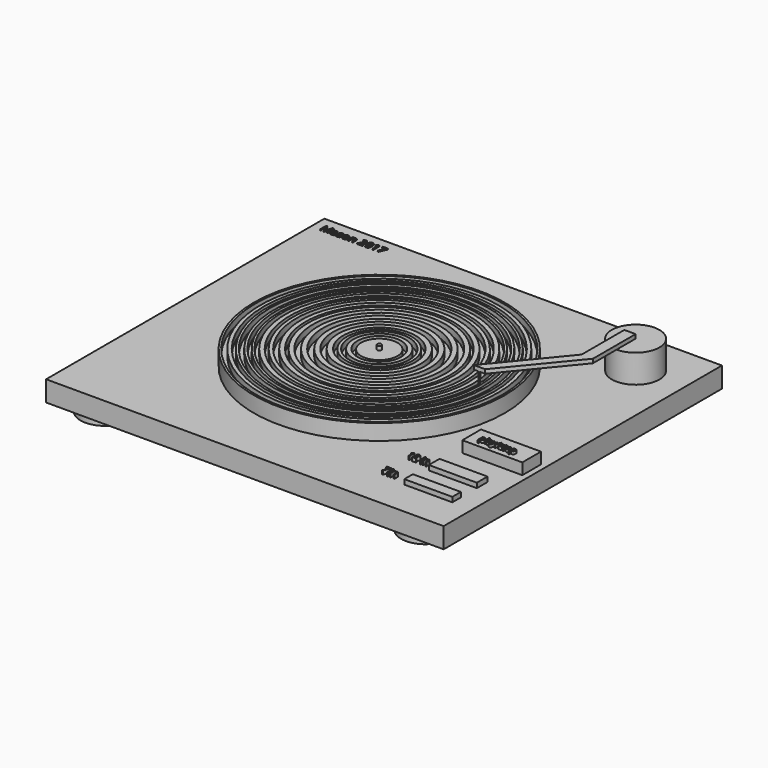
from build123d import *

# Parameters (mm, degrees)
F0_W            = 98.6984670162
F0_H            = 86.3612965102
F1_DEPTH        = 5.08
F2_R            = 31.156005255
F3_DEPTH        = 2.3
F4_R            = 31.156005255
F4_R_2          = 30.6611592983
F4_R_3          = 29.4866578201
F4_R_4          = 28.6056057905
F4_R_5          = 27.8142144613
F4_R_6          = 27.2510988872
F4_R_7          = 26.1923924199
F4_R_8          = 25.5781961877
F4_R_9          = 24.7586671221
F4_R_10         = 24.2262392051
F4_R_11         = 23.29553032
F4_R_12         = 22.2252370843
F4_R_13         = 21.4545488022
F4_R_14         = 20.5897211573
F4_R_15         = 19.4222273733
F4_R_16         = 18.2918713325
F4_R_17         = 17.6011317981
F4_R_18         = 16.4888289816
F4_R_19         = 15.1890669019
F4_R_20         = 13.9911540863
F4_R_21         = 12.6250610934
F4_R_22         = 11.4428912901
F4_R_23         = 10.2118226797
F4_R_24         = 8.9722442964
F4_R_25         = 8.1242020252
F4_R_26         = 7.4171270481
F4_R_27         = 6.4477778527
F4_R_28         = 5.420549124
F5_DEPTH        = 1.6
F6_R            = 5.9132088967
F7_DEPTH        = 7
F9_DEPTH        = 1
F11_DEPTH       = 0.4
F12_R           = 4.5011682677
F13_DEPTH       = 1.5
F14_R           = 0.5209758674
F15_DEPTH       = 1
F16_R           = 6
F17_DEPTH       = 2.6
F18_W           = 11.9140781462
F18_H           = 3.3094678074
F18_H_2         = 2.6475712657
F19_DEPTH       = 1.2
F20_TEXT_SIZE   = 2.5280596068
F20_TEXT_SIZE_2 = 2.2982376524
F21_DEPTH       = 0.9
F22_W           = 14.8925930262
F22_H           = 5.7915654033
F23_DEPTH       = 2.8
F24_TEXT_SIZE   = 2.0432040199
F25_DEPTH       = 0.7
F26_TEXT_SIZE   = 2.7578841481
F27_DEPTH       = 0.2


# Not quite as in the source:
# - Text() gives the source's letters only with a copy of the font that has no kerning and outlines rounded to 1/6400 em; it was checked with that copy


with BuildPart() as f1:
    # F0 (on Top) → F1 (new body)
    with BuildSketch(Plane.XY):
        with Locations((2.190053463, -1.2775995013)):
            Rectangle(F0_W, F0_H)
    extrude(amount=F1_DEPTH)

    # F2 (on face) → F3 (join)
    with BuildSketch(Plane.XY.offset(5.08)):
        Circle(F2_R)
    extrude(amount=F3_DEPTH)

    # F4 (on face) → F5 (join)
    with BuildSketch(Plane.XY.offset(7.38)):
        Circle(F4_R)
        Circle(F4_R_2, mode=Mode.SUBTRACT)
        Circle(F4_R_3)
        Circle(F4_R_4, mode=Mode.SUBTRACT)
        Circle(F4_R_5)
        Circle(F4_R_6, mode=Mode.SUBTRACT)
        Circle(F4_R_7)
        Circle(F4_R_8, mode=Mode.SUBTRACT)
        Circle(F4_R_9)
        Circle(F4_R_10, mode=Mode.SUBTRACT)
        Circle(F4_R_11)
        Circle(F4_R_12, mode=Mode.SUBTRACT)
        Circle(F4_R_13)
        Circle(F4_R_14, mode=Mode.SUBTRACT)
        Circle(F4_R_15)
        Circle(F4_R_16, mode=Mode.SUBTRACT)
        Circle(F4_R_17)
        Circle(F4_R_18, mode=Mode.SUBTRACT)
        Circle(F4_R_19)
        Circle(F4_R_20, mode=Mode.SUBTRACT)
        Circle(F4_R_21)
        Circle(F4_R_22, mode=Mode.SUBTRACT)
        Circle(F4_R_23)
        Circle(F4_R_24, mode=Mode.SUBTRACT)
        Circle(F4_R_25)
        Circle(F4_R_26, mode=Mode.SUBTRACT)
        Circle(F4_R_27)
        Circle(F4_R_28, mode=Mode.SUBTRACT)
    extrude(amount=F5_DEPTH)

    # F6 (on face) → F7 (join)
    with BuildSketch(Plane.XY.offset(5.08)):
        with Locations((39.8352257907, 29.7486409545)):
            Circle(F6_R)
    extrude(amount=F7_DEPTH)

    # F8 (on face) → F9 (join)
    with BuildSketch(Plane.XY.offset(12.08)):
        with BuildLine():
            Line((39.8352257907, 16.5107790381), (39.8352257907, 23.8354320578))
            ThreePointArc((39.8352257907, 23.8354320578), (38.3920917226, 24.0142357092), (37.0362326503, 24.5398333313))
            Line((37.0362326503, 24.5398333313), (37.0362326503, 16.5107790381))
            Line((37.0362326503, 16.5107790381), (23.4674233943, 0))
            Line((23.4674233943, 0), (26.2664165348, 0))
            Line((26.2664165348, 0), (39.8352257907, 16.5107790381))
        make_face()
        with BuildLine():
            Line((39.8352257907, 23.8354320578), (39.8352257907, 29.7486409545))
            Line((39.8352257907, 29.7486409545), (37.0362326503, 29.7486409545))
            Line((37.0362326503, 29.7486409545), (37.0362326503, 24.5398333313))
            ThreePointArc((37.0362326503, 24.5398333313), (38.3920917226, 24.0142357092), (39.8352257907, 23.8354320578))
        make_face()
    extrude(amount=F9_DEPTH)

    # F12 (on face) → F13 (join)
    with BuildSketch(Plane.XY.offset(7.38)):
        Circle(F12_R)
    extrude(amount=F13_DEPTH)

    # F14 (on face) → F15 (join)
    with BuildSketch(Plane.XY.offset(8.88)):
        Circle(F14_R)
    extrude(amount=F15_DEPTH)

    # F16 (on face) → F17 (join)
    with BuildSketch(Plane(origin=(0, 0, 0), x_dir=(1, 0, 0), z_dir=(0, 0, -1))):
        with Locations((-39.0016975826, 36.4318301551)):
            Circle(F16_R)
        with Locations((40.5705314347, 36.4318301551)):
            Circle(F16_R)
        with Locations((40.5705314347, -31.0741129819)):
            Circle(F16_R)
        with Locations((-39.0016975826, -32.8677496754)):
            Circle(F16_R)
    extrude(amount=F17_DEPTH)

    # F18 (on face) → F19 (join)
    with BuildSketch(Plane.XY.offset(5.08)):
        with Locations((40.6625922769, -26.3468036428)):
            Rectangle(F18_W, F18_H)
        with Locations((40.6625922769, -34.2895202339)):
            Rectangle(F18_W, F18_H_2)
    extrude(amount=F19_DEPTH)

    # F20 (on face) → F21 (join)
    with BuildSketch(Plane.XY.offset(5.08)):
        with Locations((28.2520949841, -34.9514111876)):
            Text('7in', F20_TEXT_SIZE, font='Open Sans', text_align=(TextAlign.LEFT, TextAlign.BOTTOM))
        with Locations((28.2520949841, -27.0086936653)):
            Text('12 in', F20_TEXT_SIZE_2, font='Open Sans', text_align=(TextAlign.LEFT, TextAlign.BOTTOM))
    extrude(amount=F21_DEPTH)

    # F22 (on face) → F23 (join)
    with BuildSketch(Plane.XY.offset(5.08)):
        with Locations((42.6482707262, -15.3428288177)):
            Rectangle(F22_W, F22_H)
    extrude(amount=F23_DEPTH)

    # F24 (on face) → F25 (join)
    with BuildSketch(Plane.XY.offset(7.88)):
        with Locations((38.0816571414, -16.813935712)):
            Text('play/stop', F24_TEXT_SIZE, font='Open Sans', text_align=(TextAlign.LEFT, TextAlign.BOTTOM))
    extrude(amount=F25_DEPTH)

    # F26 (on face) → F27 (join)
    with BuildSketch(Plane.XY.offset(5.08)):
        with Locations((-45.0525693595, 37.5258885324)):
            Text('Mason 2017', F26_TEXT_SIZE, font='Open Sans', text_align=(TextAlign.LEFT, TextAlign.BOTTOM))
    extrude(amount=F27_DEPTH)


with BuildPart() as f11:
    # F10 (on face) → F11 (new body)
    with BuildSketch(Plane.XZ):
        Polygon((24.653095752, 8.9536914602), (24.8669199646, 12.08), (24.653095752, 12.08), align=None)
    extrude(amount=-F11_DEPTH)


solid = Compound([f1.part, f11.part])
